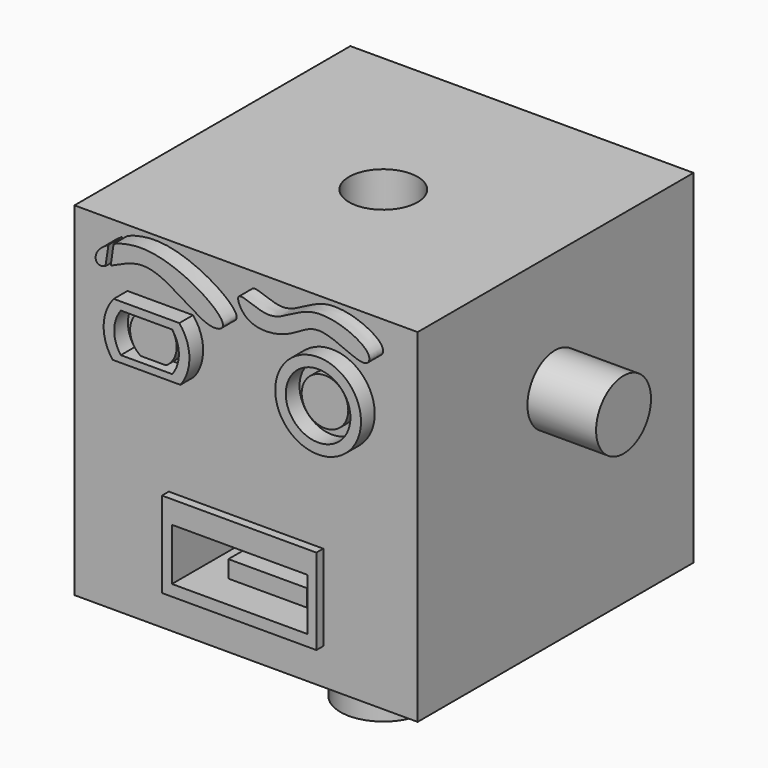
from build123d import *

# Parameters (mm, degrees)
F0_W          = 20
F0_H          = 20
F1_DEPTH      = 10
F1_DEPTH_BACK = 10.1
F3_R          = 2.5
F4_DEPTH      = 6
F5_R          = 2
F6_DEPTH      = 4
F8_DEPTH      = 1
F2_R          = 2.5
F2_R_2        = 1.8839772237
F9_DEPTH      = 1
F10_R         = 1.3573701911
F11_DEPTH     = 0.5
F12_W         = 9
F12_H         = 5
F12_W_2       = 7.9026320018
F12_H_2       = 3.0369618908
F13_DEPTH     = 0.5
F14_DEPTH     = 5
F15_W         = 4.5965062454
F15_H         = 2.9658381827
F16_DEPTH     = 1
F17_R         = 2
F18_DEPTH     = 10


# Not quite as in the source:
# - a pattern or mirror of a feature is missing from the dataset's text; its kind, count and spacing are read off the source's solid


with BuildPart() as f1:
    # F0 (on Front) → F1 (new body, two sides)
    with BuildSketch(Plane.XZ) as f1_sk:
        Rectangle(F0_W, F0_H)
    extrude(amount=F1_DEPTH)
    extrude(f1_sk.sketch, amount=-F1_DEPTH_BACK)

    # F3 (on face) → F4 (join)
    with BuildSketch(Plane(origin=(0, 0, -10), x_dir=(1, 0, 0), z_dir=(0, 0, -1))):
        Circle(F3_R)
    extrude(amount=F4_DEPTH)

    # F5 (on face) → F6 (join)
    with BuildSketch(Plane.YZ.offset(10)):
        with Locations((0, 3.0001785737)):
            Circle(F5_R)
    f6 = extrude(amount=F6_DEPTH)

    # F6_copies: F6 across plane
    add(f6.mirror(Plane(origin=(0, 0, 0), x_dir=(0, 0, -1), z_dir=(-1, 0, 0))))

    # F7 (on face) → F8 (join)
    with BuildSketch(Plane.XZ.offset(10)):
        with BuildLine():
            add(Edge.make_bspline(
                [(7.7260467224, 8.0762784928), (7.2086697911, 7.9845892861), (4.9588884294, 9.5225004004), (3.4008396285, 7.8448789895), (0.7688019503, 7.6559223164), (-0.0428373735, 9.6922571059), (2.4742152448, 8.0528779948), (4.479723086, 10.4981199234), (8.2903261876, 8.9052336103), (7.9607643979, 8.1178750082), (7.7260467224, 8.0762784928)],
                knots=[0, 0, 0, 0, 0.145679393, 0.2746377747, 0.411140374, 0.5029732293, 0.6216284586, 0.7721347563, 0.9339098317, 1, 1, 1, 1], degree=3))
        make_face()
        with BuildLine():
            Line((-7.3962743957, 8.130105928), (-7.2186427029, 9.2839803847))
            add(Edge.make_bspline(
                [(-7.2186427029, 9.2839803847), (-7.5895724, 9.076773158), (-8.1085460348, 8.5639491599), (-7.9332602241, 8.1095149337), (-7.7260467224, 8.0762784928)],
                knots=[0.8450356741, 0.8450356741, 0.8450356741, 0.8450356741, 0.9208330932, 1, 1, 1, 1], degree=3))
            add(Edge.make_bspline(
                [(-7.7260467224, 8.0762784928), (-7.636698412, 8.0619472846), (-7.5254733116, 8.0846003978), (-7.3962743957, 8.130105928)],
                knots=[0, 0, 0, 0, 0.0341359482, 0.0341359482, 0.0341359482, 0.0341359482], degree=3))
        make_face()
        with BuildLine():
            add(Edge.make_bspline(
                [(-7.0876194027, 8.2600987876), (-6.5687825393, 8.5013247619), (-4.569681637, 9.6142581743), (-1.738561118, 6.6882346812), (0.3741280236, 7.3787117351), (-3.8767286459, 10.1353693076), (-6.3621761685, 9.667824135), (-6.919334154, 9.4302727567)],
                knots=[0.0589433384, 0.0589433384, 0.0589433384, 0.0589433384, 0.1745038212, 0.3926307023, 0.4916975866, 0.7270488643, 0.8260908422, 0.8260908422, 0.8260908422, 0.8260908422], degree=3))
            Line((-6.919334154, 9.4302727567), (-7.0876194027, 8.2600987876))
        make_face()
    extrude(amount=F8_DEPTH)

    # F2 (on face) → F9 (join)
    with BuildSketch(Plane.XZ.offset(10)):
        with Locations((5, 5)):
            Circle(F2_R)
        with Locations((5, 5)):
            Circle(F2_R_2, mode=Mode.SUBTRACT)
        with BuildLine():
            Line((-5.9748485127, 6.6121540115), (-6.9107483987, 6.6121540115))
            ThreePointArc((-6.9107483987, 6.6121540115), (-7.4995103565, 5.0494770438), (-6.9730508021, 3.464724607))
            Line((-6.9730508021, 3.464724607), (-6.0919247442, 3.464724607))
            Line((-6.0919247442, 3.464724607), (-3.9080752558, 3.464724607))
            Line((-3.9080752558, 3.464724607), (-3.0269491979, 3.464724607))
            ThreePointArc((-3.0269491979, 3.464724607), (-2.5004896435, 5.0494770438), (-3.0892516013, 6.6121540115))
            Line((-3.0892516013, 6.6121540115), (-4.0251514873, 6.6121540115))
            Line((-4.0251514873, 6.6121540115), (-5.9748485127, 6.6121540115))
        make_face()
        with BuildLine():
            ThreePointArc((-6.4995787818, 3.8595467319), (-6.8839712306, 5.0047520465), (-6.4938064783, 6.148003652))
            Line((-6.4938064783, 6.148003652), (-3.5061935217, 6.148003652))
            ThreePointArc((-3.5061935217, 6.148003652), (-3.1160287694, 5.0047520465), (-3.5004212182, 3.8595467319))
            Line((-3.5004212182, 3.8595467319), (-6.4995787818, 3.8595467319))
        make_face(mode=Mode.SUBTRACT)
    extrude(amount=F9_DEPTH)

    # F10 (on face) → F11 (join)
    with BuildSketch(Plane.XZ.offset(10)):
        with Locations((5, 5)):
            Circle(F10_R)
        with Locations((-5, 5)):
            Circle(F10_R)
    extrude(amount=F11_DEPTH)

    # F12 (on face) → F13 (join)
    with BuildSketch(Plane.XZ.offset(10)):
        with Locations((0, -5.3983260319)):
            Rectangle(F12_W, F12_H)
        with Locations((0.0326556619, -5.7267351076)):
            Rectangle(F12_W_2, F12_H_2, mode=Mode.SUBTRACT)
    extrude(amount=F13_DEPTH)

    # F14 (cut): a face of the model
    f14_faces = [f1.faces().sort_by_distance(p)[0] for p in [
        (0.0326556619, -10, -5.7267351076),
    ]]
    extrude(f14_faces, amount=-F14_DEPTH, mode=Mode.SUBTRACT)

    # F15 (on face) → F16 (join)
    with BuildSketch(Plane.XY.offset(-7.245216053)):
        with Locations((0.0545033254, -7.0004777517)):
            Rectangle(F15_W, F15_H)
    extrude(amount=F16_DEPTH)

    # F17 (on face) → F18 (cut)
    with BuildSketch(Plane.XY.offset(10)):
        Circle(F17_R)
    extrude(amount=-F18_DEPTH, mode=Mode.SUBTRACT)


solid = f1.part
